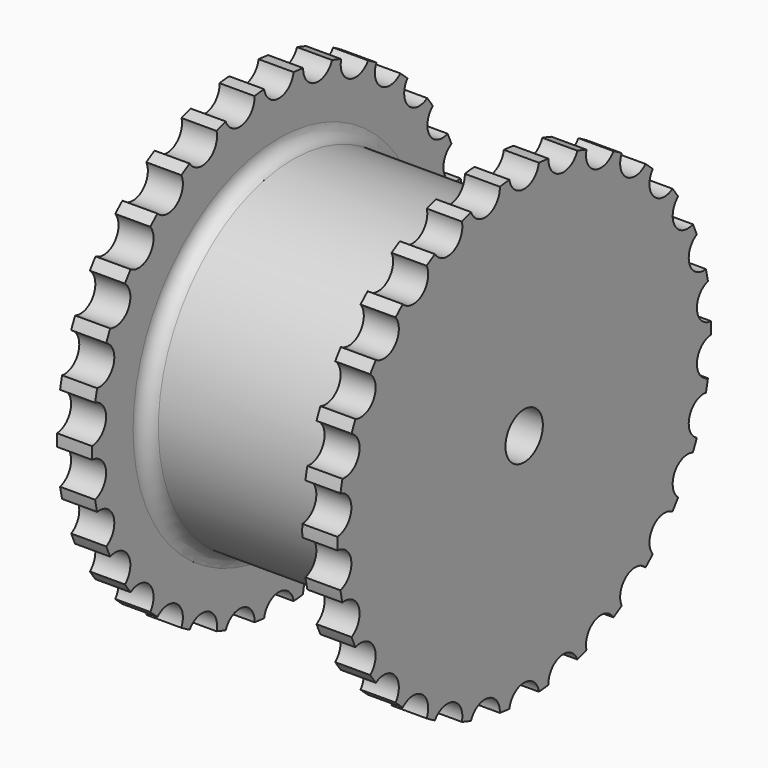
from build123d import *

# Parameters (mm, degrees)
F0_R            = 50
F1_DEPTH        = 30
F2_W            = 45
F2_H            = 14
F4_R            = 4
F5_DEPTH        = 30
F5_COPIES_COUNT = 30
F7_DEPTH        = 1.5
F7_COPIES_COUNT = 4
F8_R            = 3


# Not quite as in the source:
# - a pattern or mirror of a feature is missing from the dataset's text; its kind, count and spacing are read off the source's solid


with BuildPart() as f1:
    # F0 (on Right) → F1 (new body, symmetric)
    with BuildSketch(Plane.YZ):
        Circle(F0_R)
    extrude(amount=F1_DEPTH, both=True)

    # F2 (on Front) → F3 (revolve, cut)
    with BuildSketch(Plane.XZ):
        with Locations((0, 43)):
            Rectangle(F2_W, F2_H)
        Polygon((-30, 0), (23, 0), (30, 0), (30, 5), (23, 5), (10, 5), (10, 10), (23, 10), (23, 27.5), (-30, 27.5), align=None)
    revolve(axis=Axis((39.8031175137, 0, 0), (1, 0, 0)), mode=Mode.SUBTRACT)

    # F4 (on Right) → F5 (cut, symmetric)
    with BuildSketch(Plane.YZ):
        with Locations((0, 50.5)):
            Circle(F4_R)
    f5 = extrude(amount=F5_DEPTH, both=True, mode=Mode.SUBTRACT)

    # F5_copies: F5 ×30 about axis
    f5_copies_axis = Axis((0, 0, 0), (1, 0, 0))
    for i in range(1, F5_COPIES_COUNT):
        add(f5.rotate(f5_copies_axis, i * 360 / F5_COPIES_COUNT), mode=Mode.SUBTRACT)

    # F6 (on Front) → F7 (join, symmetric)
    with BuildSketch(Plane.XZ):
        Polygon((-30, 27.5), (10.4571428571, 9.8), (23, 9.8), (23, 27.5), align=None)
    f7 = extrude(amount=F7_DEPTH, both=True)

    # F7_copies: F7 ×4 about axis
    f7_copies_axis = Axis((0, 0, 0), (1, 0, 0))
    for i in range(1, F7_COPIES_COUNT):
        add(f7.rotate(f7_copies_axis, i * 360 / F7_COPIES_COUNT))

    # F8
    f8_edges = [f1.edges().sort_by_distance(p)[0] for p in [
        (22.5, 0, -36),
        (-22.5, 0, -36),
    ]]
    fillet(f8_edges, radius=F8_R)


solid = f1.part
